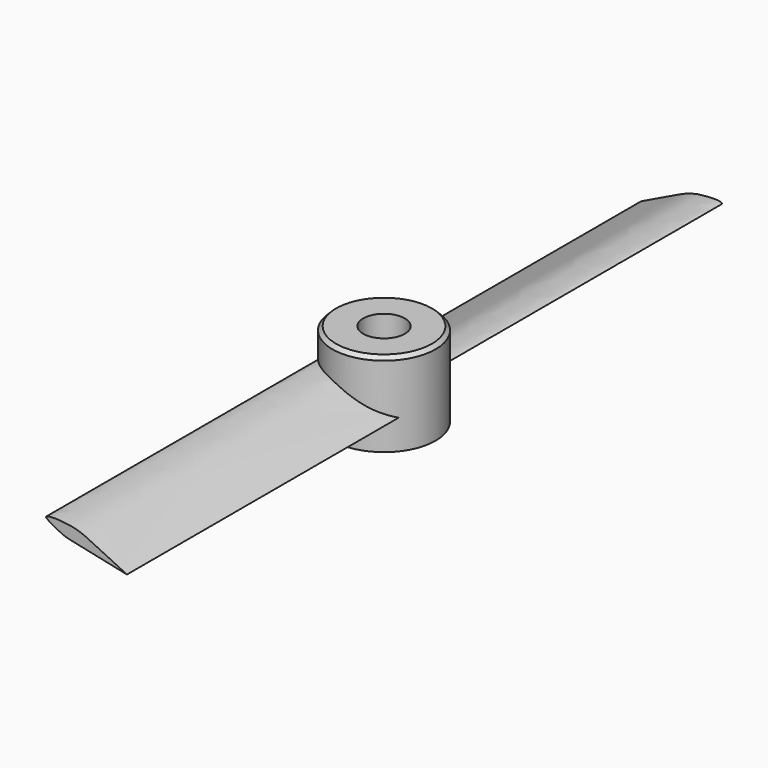
from build123d import *

# Parameters (mm, degrees)
F0_R     = 7.05
F0_R_2   = 2.85
F1_DEPTH = 11.5
F3_DEPTH = 50.8
F4_R     = 5
F6_DEPTH = 50.8
F7_R     = 5
F8_DEPTH = 25
F9_SIZE  = 0.5


# Not quite as in the source:
# - a feature names something its author has since deleted; it is built from what else it names


with BuildPart() as f1:
    # F0 (on Top) → F1 (new body)
    with BuildSketch(Plane.XY):
        Circle(F0_R)
        Circle(F0_R_2, mode=Mode.SUBTRACT)
        Circle(F0_R_2)
    extrude(amount=F1_DEPTH)

    # F2 (on Front) → F3 (join)
    with BuildSketch(Plane.XZ):
        with BuildLine():
            add(Edge.make_bspline(
                [(-3.1119612486, 5.9019833995), (-4.352930456, 6.6519015813), (-6.9311743253, 7.7158918454), (-2.3785587972, 7.6153860853), (-0.2352237379, 6.910360475), (2.7021392414, 5.4029427526), (4.5777539416, 4.5069045056), (5.5192211105, 4.0626041336)],
                knots=[0, 0, 0, 0, 0.1977876363, 0.3919769243, 0.5835513721, 0.7917756861, 1, 1, 1, 1], degree=3))
            Line((-3.1119612486, 5.9019833995), (5.5192211105, 4.0626041336))
        make_face()
    extrude(amount=F3_DEPTH)

    # F4
    f4_edges = [f1.edges().sort_by_distance(p)[0] for p in [
        (-3.111961, -28.562997, 5.901983),
    ]]
    fillet(f4_edges, radius=F4_R)

    # F5 (on Front) → F6 (join)
    with BuildSketch(Plane.XZ):
        with BuildLine():
            Line((-5.5194998324, 4.0625152563), (3.1116825268, 5.9018945222))
            add(Edge.make_bspline(
                [(3.1116825268, 5.9018945222), (4.3526517342, 6.651812704), (6.9308956034, 7.7158029681), (2.3782800753, 7.615297208), (0.2349450161, 6.9102715977), (-2.7024179633, 5.4028538753), (-4.5780326634, 4.5068156283), (-5.5194998324, 4.0625152563)],
                knots=[0, 0, 0, 0, 0.1977876363, 0.3919769243, 0.5835513721, 0.7917756861, 1, 1, 1, 1], degree=3))
        make_face()
    extrude(amount=-F6_DEPTH)

    # F7
    f7_edges = [f1.edges().sort_by_distance(p)[0] for p in [
        (3.111683, 28.563065, 5.901895),
    ]]
    fillet(f7_edges, radius=F7_R)

    # F0 (on Top) → F8 (cut)
    with BuildSketch(Plane.XY):
        Circle(F0_R_2)
    extrude(amount=F8_DEPTH, mode=Mode.SUBTRACT)

    # F9
    f9_edges = [f1.edges().sort_by_distance(p)[0] for p in [
        (-7.05, 0, 11.5),
    ]]
    chamfer(f9_edges, length=F9_SIZE)


solid = f1.part
